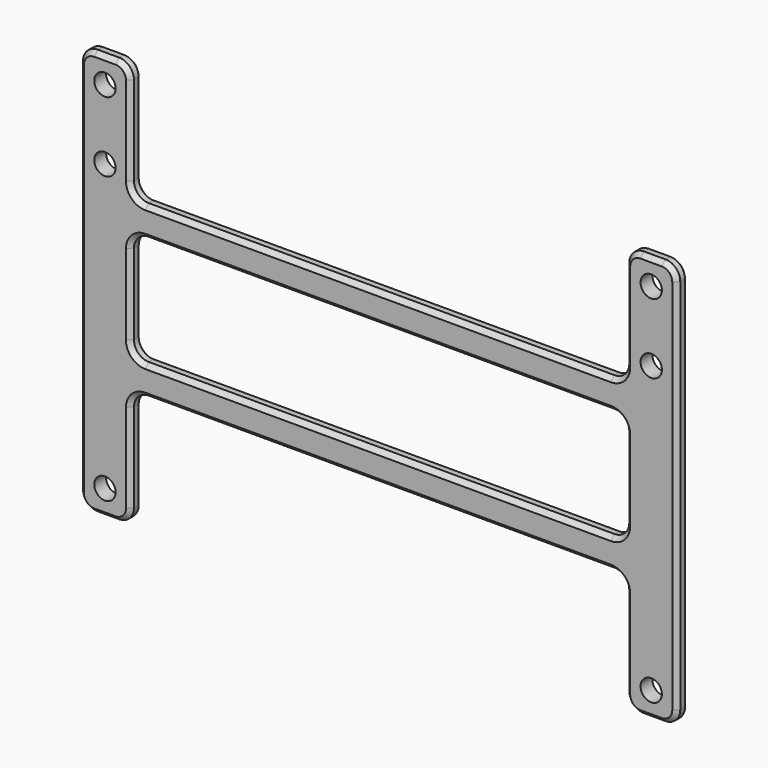
from build123d import *

# Parameters (mm, degrees)
F0_W     = 0.0285906434
F0_H     = 5
F0_W_2   = 41.8
F0_R     = 1.8
F1_DEPTH = 2.5
F2_R     = 2.5
F3_SIZE  = 0.75


# Not quite as in the source:
# - a feature names something its author has since deleted; it is built from what else it names


with BuildPart() as f1:
    # F0 (on Front) → F1 (new body)
    with BuildSketch(Plane.XZ):
        with Locations((-41.8142953217, 18.525)):
            Rectangle(F0_W, F0_H)
        with Locations((41.8142953217, 18.525)):
            Rectangle(F0_W, F0_H)
        with Locations((-20.9, 18.525)):
            Rectangle(F0_W_2, F0_H)
        with Locations((20.9, 18.525)):
            Rectangle(F0_W_2, F0_H)
        with Locations((20.9, 42.125)):
            Rectangle(F0_W_2, F0_H)
        Polygon((41.8, 64.625), (41.8, 44.625), (41.8, 39.625), (41.8, 21.025), (41.8285906434, 21.025), (41.8285906434, 16.025), (41.8, 16.025), (41.8, -3.975), (50.4, -3.975), (50.4, 64.625), align=None)
        with Locations((46.1, 0.325)):
            Circle(F0_R, mode=Mode.SUBTRACT)
        with Locations((46.1, 48.525)):
            Circle(F0_R, mode=Mode.SUBTRACT)
        with Locations((46.1, 60.325)):
            Circle(F0_R, mode=Mode.SUBTRACT)
        with Locations((-20.9, 42.125)):
            Rectangle(F0_W_2, F0_H)
        Polygon((-41.8, 64.625), (-50.4, 64.625), (-50.4, -3.975), (-41.8, -3.975), (-41.8, 16.025), (-41.8285906434, 16.025), (-41.8285906434, 21.025), (-41.8, 21.025), (-41.8, 39.625), (-41.8, 44.625), align=None)
        with Locations((-46.1, 0.325)):
            Circle(F0_R, mode=Mode.SUBTRACT)
        with Locations((-46.1, 48.525)):
            Circle(F0_R, mode=Mode.SUBTRACT)
        with Locations((-46.1, 60.325)):
            Circle(F0_R, mode=Mode.SUBTRACT)
    extrude(amount=F1_DEPTH)

    # F2
    f2_edges = [f1.edges().sort_by_distance(p)[0] for p in [
        (-41.8, -1.25, 44.625),
        (41.8, -1.25, 44.625),
        (-41.8, -1.25, 39.625),
        (41.8, -1.25, 39.625),
        (-41.8, -1.25, 21.025),
        (41.8, -1.25, 21.025),
        (-41.8, -1.25, 16.025),
        (41.8, -1.25, 16.025),
        (41.8, -1.25, -3.975),
        (50.4, -1.25, -3.975),
        (-50.4, -1.25, -3.975),
        (-41.8, -1.25, -3.975),
        (50.4, -1.25, 64.625),
        (41.8, -1.25, 64.625),
        (-50.4, -1.25, 64.625),
        (-41.8, -1.25, 64.625),
    ]]
    fillet(f2_edges, radius=F2_R)

    # F3
    f3_edges = [f1.edges().sort_by_distance(p)[0] for p in [
        (0, 0, 16.025),
        (0, 0, 39.625),
        (-46.1, -2.5, 64.625),
        (0, -2.5, 39.625),
    ]]
    chamfer(f3_edges, length=F3_SIZE)


solid = f1.part
